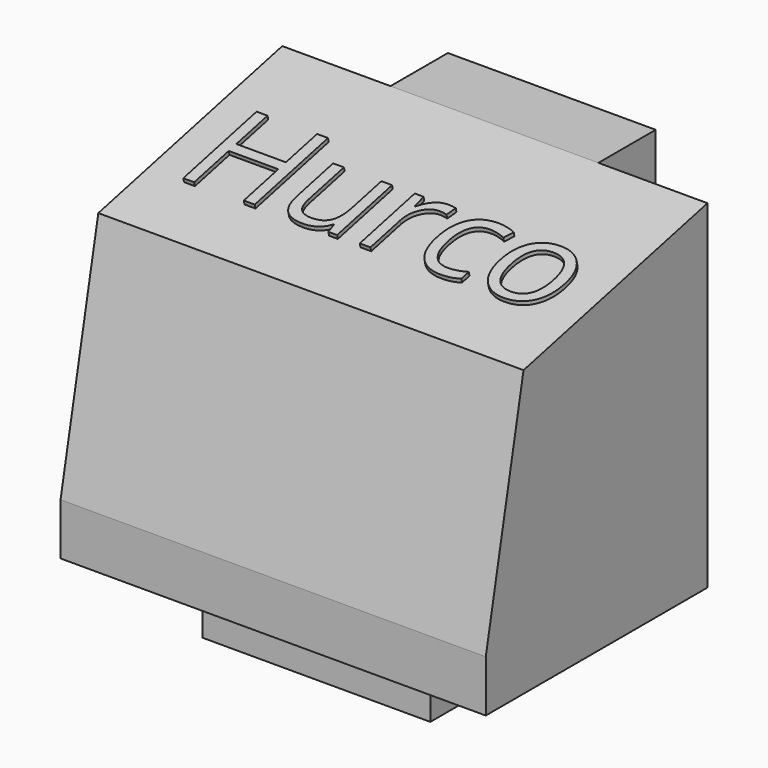
from build123d import *

# Parameters (mm, degrees)
F1_DEPTH     = 2500
F3_DEPTH     = 2670.001
F4_TEXT_SIZE = 827.3717429903
F5_DEPTH     = 25
F7_DEPTH     = 375


# Not quite as in the source:
# - Text() gives the source's letters only with a copy of the font that has no kerning and outlines rounded to 1/6400 em; it was checked with that copy


with BuildPart() as f1:
    # F0 (on Top) → F1 (new body)
    with BuildSketch(Plane.XY):
        Polygon((0, 1740), (0, 0), (2670, 0), (2670, 1740), (1985, 1740), (1985, 2190), (680, 2190), (680, 1740), align=None)
    extrude(amount=F1_DEPTH)

    # F2 (on face) → F3 (cut, through all)
    with BuildSketch(Plane.YZ.offset(2670)):
        Polygon((0, 2500), (0, 700), (296.4625060558, 2163.7206792831), (1740, 2500), align=None)
    extrude(amount=-F3_DEPTH, mode=Mode.SUBTRACT)

    # F4 (on face) → F5 (join)
    with BuildSketch(Plane(origin=(0, -462.8435598764, 1986.836511647), x_dir=(1, 0, 0), z_dir=(0, -0.2268801868, 0.973922677))):
        with Locations((149.3750363588, 1174.4294166565)):
            Text('Hurco', F4_TEXT_SIZE, font='Open Sans', text_align=(TextAlign.LEFT, TextAlign.BOTTOM))
    extrude(amount=F5_DEPTH)

    # F6 (on face) → F7 (cut)
    with BuildSketch(Plane(origin=(0, 0, 0), x_dir=(1, 0, 0), z_dir=(0, 0, -1))):
        Polygon((0, 0), (0, -1740), (620, -1740), (620, -340), (2050, -340), (2050, -1740), (2670, -1740), (2670, 0), align=None)
    extrude(amount=-F7_DEPTH, mode=Mode.SUBTRACT)


solid = f1.part
